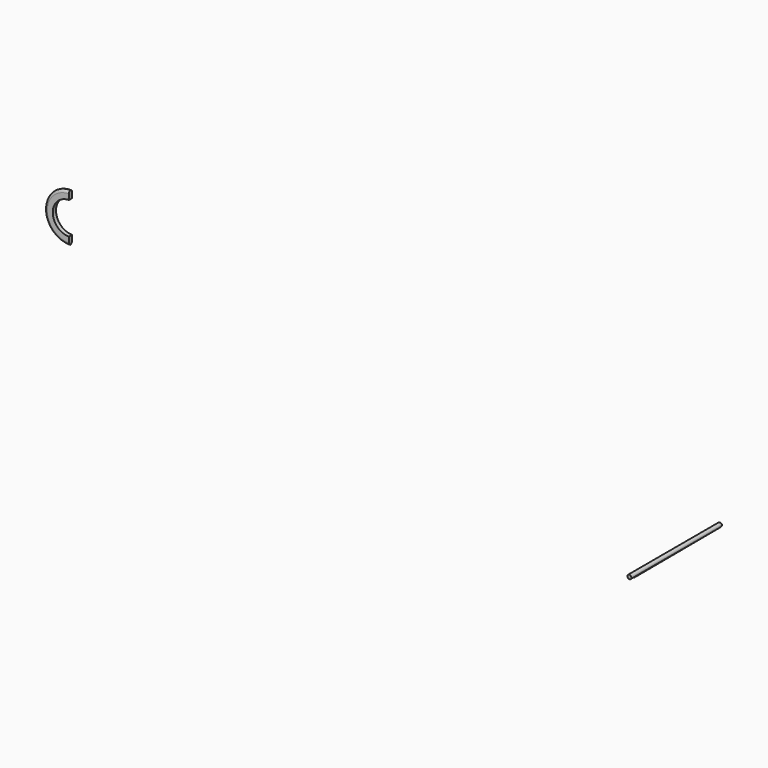
from build123d import *

# Parameters (mm, degrees)
F0_R          = 0.1984375
F1_DEPTH      = 11.1125
F6_DEPTH      = 0.1984375
F6_DEPTH_BACK = 0.1984375
F7_T2_ANGLE   = 210.6068917121
F7_T4_ANGLE   = 210.6068917121


# Not quite as in the source:
# - a fillet or chamfer that OpenCascade refuses, or shapes differently, is made with other operations: its cross-section is extruded or revolved along the edge and cut away or added


with BuildPart() as f1:
    # F0 (on Front) → F1 (new body)
    with BuildSketch(Plane.XZ):
        Circle(F0_R)
    extrude(amount=F1_DEPTH)

    # F2 (on Front) → F3 (revolve)
    with BuildSketch(Plane.XZ):
        Polygon((-8.5126688742, -7.1429773126), (0, 0), (-0.1267016231, 0.1509971145), (-8.6393704972, -6.9919801982), align=None)
    revolve(axis=Axis((-4.2563344371, 0, -3.5714886563), (-0.7660444431, 0, -0.6427876097)))

    # F4 (on face) → F5 (revolve)
    with BuildSketch(Plane(origin=(0, 0, 0), x_dir=(-1, 0, 0), z_dir=(0, 1, 0))):
        with BuildLine():
            ThreePointArc((-0.1984375, 0), (-0.1802970974, -0.0828878645), (-0.129192543, -0.1506211414))
            Line((-0.129192543, -0.1506211414), (0.1272588737, 0.1522584003))
            ThreePointArc((0.1272588737, 0.1522584003), (-0.0840372199, 0.1797642542), (-0.1984375, 0))
        make_face()
    revolve(axis=Axis((0.0009668347, 0, 0.0008186295), (-0.6461899668, 0, 0.7631766027)))


with BuildPart() as f6:
    # F2 (on Front) → F6 (new body, two sides)
    with BuildSketch(Plane.XZ) as f6_sk:
        with BuildLine():
            Line((-64.0807822347, 7.4859789066), (-64.0807822347, 8.2797289066))
            ThreePointArc((-64.0807822347, 8.2797289066), (-66.4620322347, 5.8984789066), (-64.0807822347, 3.5172289066))
            Line((-64.0807822347, 3.5172289066), (-64.0807822347, 4.3109789066))
            ThreePointArc((-64.0807822347, 4.3109789066), (-65.6682822347, 5.8984789066), (-64.0807822347, 7.4859789066))
        make_face()
    extrude(amount=F6_DEPTH)
    extrude(f6_sk.sketch, amount=-F6_DEPTH_BACK)

    # F7: fillet of radius 0.254 on 2 edges, made by hand

    # F7_s1 → F7_t2 (revolve, cut)
    with BuildSketch(Plane(origin=(-61.1185306696, 0, 16.7240888712), x_dir=(0, 1, 0), z_dir=(0.964541547, 0, -0.2639310595))):
        with BuildLine():
            ThreePointArc((0.0555625, -8.8423307762), (-0.1240426224, -8.9167256538), (-0.1984375, -9.0963307762))
            Line((-0.1984375, -9.0963307762), (-0.1984375, -8.8423307762))
            Line((-0.1984375, -8.8423307762), (0.0555625, -8.8423307762))
        make_face()
    revolve(axis=Axis((-64.0807822347, -0.1984375, 5.8984789066), (0, -1, 0)), revolution_arc=F7_T2_ANGLE, mode=Mode.SUBTRACT)

    # F7_s3 → F7_t4 (revolve, cut)
    with BuildSketch(Plane(origin=(-61.1185306696, 0, 16.7240888712), x_dir=(0, 1, 0), z_dir=(0.964541547, 0, -0.2639310595))):
        with BuildLine():
            ThreePointArc((0.1984375, -9.0963307762), (0.1240426224, -8.9167256538), (-0.0555625, -8.8423307762))
            Line((-0.0555625, -8.8423307762), (0.1984375, -8.8423307762))
            Line((0.1984375, -8.8423307762), (0.1984375, -9.0963307762))
        make_face()
    revolve(axis=Axis((-64.0807822347, 0.1984375, 5.8984789066), (0, -1, 0)), revolution_arc=F7_T4_ANGLE, mode=Mode.SUBTRACT)


solid = Compound([f1.part, f6.part])
